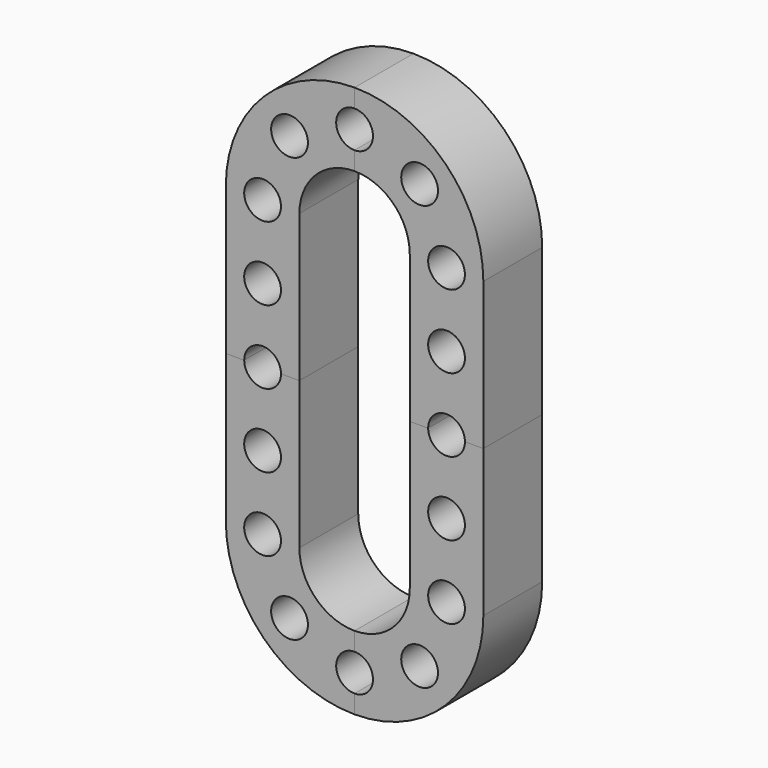
from build123d import *
from build123d import SkipClean  # not in build123d's __all__

# Parameters (mm, degrees)
F0_R     = 5
F1_DEPTH = 20


with BuildPart() as f1:
    # F0 (on Front) → F1 (new body)
    with BuildSketch(Plane.XZ):
        with BuildLine():
            ThreePointArc((-15, 40), (-10.6066017178, 50.6066017178), (0, 55))
            Line((0, 55), (0, 60))
            ThreePointArc((0, 60), (-5, 65), (0, 70))
            Line((0, 70), (0, 75))
            ThreePointArc((0, 75), (-24.7487373415, 64.7487373415), (-35, 40))
            Line((-35, 40), (-35, 0))
            Line((-35, 0), (-30, 0))
            ThreePointArc((-30, 0), (-25, 5), (-20, 0))
            Line((-20, 0), (-15, 0))
            Line((-15, 0), (-15, 40))
        make_face()
        with Locations((-25, 20)):
            Circle(F0_R, mode=Mode.SUBTRACT)
        with Locations((-25, 40)):
            Circle(F0_R, mode=Mode.SUBTRACT)
        with Locations((-17.6776695297, 57.6776695297)):
            Circle(F0_R, mode=Mode.SUBTRACT)
    extrude(amount=F1_DEPTH)

    # F2: F1 across plane


with BuildPart() as f1_1:
    add(f1.part, clean=False)
    with SkipClean():  # cleaning this boolean's faces spoils the solid; the shape is the same uncleaned
        add(f1.part.mirror(Plane.YZ), clean=False)

    # F3: F1 across plane


with BuildPart() as f1_2:
    add(f1_1.part, clean=False)
    with SkipClean():  # cleaning this boolean's faces spoils the solid; the shape is the same uncleaned
        add(f1_1.part.mirror(Plane.XY), clean=False)


solid = f1_2.part
